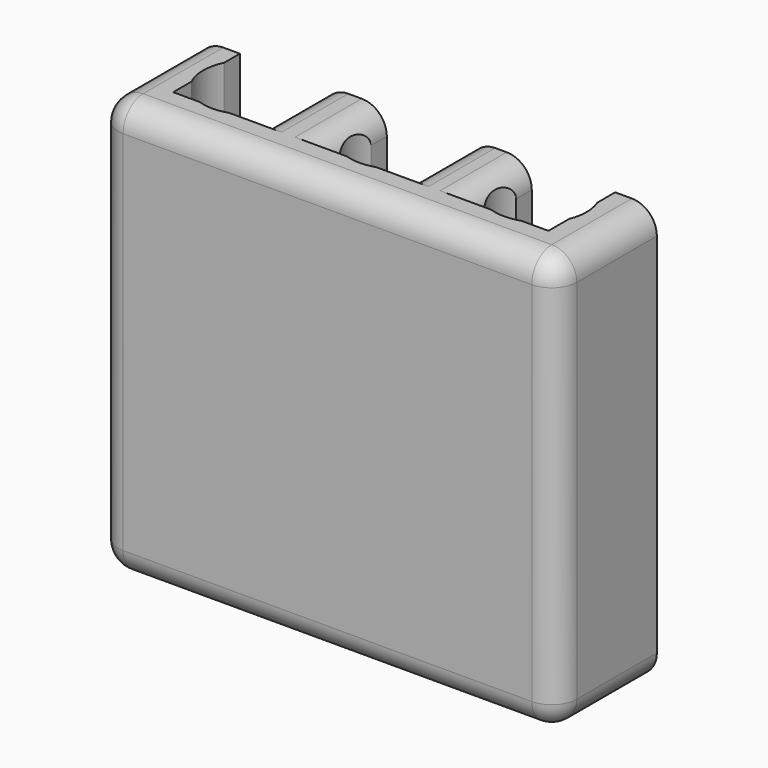
from build123d import *

# Parameters (mm, degrees)
F0_W     = 1
F0_H     = 10
F1_DEPTH = 2
F0_W_2   = 1.5239776969
F0_W_3   = 1.4760223031
F0_W_4   = 2
F2_DEPTH = 1
F3_R     = 0.6
F4_R     = 1.1
F5_DEPTH = 50


with BuildPart() as f1:
    # F0 (on Front) → F1 (new body)
    with BuildSketch(Plane.XZ):
        with Locations((-46.041754216, 24.6294103354)):
            Rectangle(F0_W, F0_H)
    extrude(amount=-F1_DEPTH)



with BuildPart() as f1b:
    # F0 (on Front) → F1, piece 2 (new body)
    with BuildSketch(Plane.XZ):
        with Locations((-42.7797653675, 24.6294103354)):
            Rectangle(F0_W_2, F0_H)
    extrude(amount=-F1_DEPTH)


with BuildPart() as f1c:
    # F0 (on Front) → F1, piece 3 (new body)
    with BuildSketch(Plane.XZ):
        with Locations((-39.2797653675, 24.6294103354)):
            Rectangle(F0_W_3, F0_H)
    extrude(amount=-F1_DEPTH)


with BuildPart() as f1d:
    # F0 (on Front) → F1, piece 4 (new body)
    with BuildSketch(Plane.XZ):
        with Locations((-36.041754216, 24.6294103354)):
            Rectangle(F0_W, F0_H)
    extrude(amount=-F1_DEPTH)


with BuildPart() as f1_1:
    add(f1.part)

    add(f1b.part)  # F2 merges F1b

    add(f1c.part)  # F2 merges F1c

    add(f1d.part)  # F2 merges F1d
    # F0 (on Front) → F2 (join)
    with BuildSketch(Plane.XZ):
        with Locations((-41.0177765191, 24.6294103354)):
            Rectangle(F0_W_4, F0_H)
        with Locations((-39.2797653675, 24.6294103354)):
            Rectangle(F0_W_3, F0_H)
        with Locations((-46.041754216, 24.6294103354)):
            Rectangle(F0_W, F0_H)
        with Locations((-44.541754216, 24.6294103354)):
            Rectangle(F0_W_4, F0_H)
        with Locations((-36.041754216, 24.6294103354)):
            Rectangle(F0_W, F0_H)
        with Locations((-42.7797653675, 24.6294103354)):
            Rectangle(F0_W_2, F0_H)
        with Locations((-37.541754216, 24.6294103354)):
            Rectangle(F0_W_4, F0_H)
    extrude(amount=F2_DEPTH)

    # F3
    f3_edges = [f1_1.edges().sort_by_distance(p)[0] for p in [
        (-43.541754, 1, 29.62941),
        (-42.017777, 1, 29.62941),
        (-40.017777, 1, 19.62941),
        (-38.541754, 1, 19.62941),
        (-40.017777, 1, 29.62941),
        (-38.541754, 1, 29.62941),
        (-43.541754, 1, 19.62941),
        (-42.017777, 1, 19.62941),
        (-46.541754, 0.5, 19.62941),
        (-46.541754, 0.5, 29.62941),
        (-35.541754, 0.5, 29.62941),
        (-41.041754, -1, 29.62941),
        (-35.541754, -1, 24.62941),
        (-46.541754, -1, 24.62941),
        (-41.041754, -1, 19.62941),
        (-35.541754, 0.5, 19.62941),
    ]]
    fillet(f3_edges, radius=F3_R)

    # F4 (on Top) → F5 (cut)
    with BuildSketch(Plane.XY):
        with Locations((-37.5576429069, 1.0389162926)):
            Circle(F4_R)
        with Locations((-41.0279254586, 1.0422003123)):
            Circle(F4_R)
        with Locations((-44.5562924673, 1.0408099828)):
            Circle(F4_R)
    extrude(amount=F5_DEPTH, mode=Mode.SUBTRACT)


solid = f1_1.part
